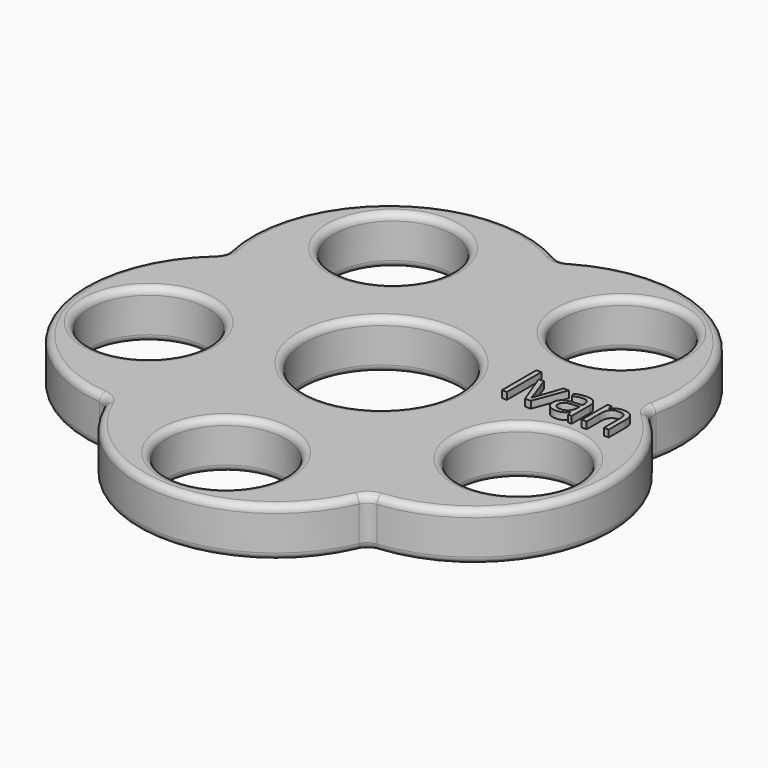
from build123d import *

# Parameters (mm, degrees)
F0_R         = 8.5
F0_R_2       = 11
F1_DEPTH     = 7
F2_R         = 2
F3_R         = 1
F4_TEXT_SIZE = 8.692171347
F5_DEPTH     = 1


# Not quite as in the source:
# - Text() gives the source's letters only with a copy of the font that has no kerning and outlines rounded to 1/6400 em; it was checked with that copy


with BuildPart() as f1:
    # F0 (on Top) → F1 (new body)
    with BuildSketch(Plane.XY):
        with BuildLine():
            ThreePointArc((30.3984422568, 9.877052624), (22.9236248394, 31.5516627806), (0, 31.9628137087))
            ThreePointArc((0, 31.9628137087), (-22.9236248394, 31.5516627806), (-30.3984422568, 9.877052624))
            ThreePointArc((-30.3984422568, 9.877052624), (-37.0912041355, -12.0516627806), (-18.7872705198, -25.8584594784))
            ThreePointArc((-18.7872705198, -25.8584594784), (0, -39), (18.7872705198, -25.8584594784))
            ThreePointArc((18.7872705198, -25.8584594784), (37.0912041355, -12.0516627806), (30.3984422568, 9.877052624))
        make_face()
        with Locations((0, -28)):
            Circle(F0_R, mode=Mode.SUBTRACT)
        with Locations((-26.6295824563, -8.6524758425)):
            Circle(F0_R, mode=Mode.SUBTRACT)
        with Locations((26.6295824563, -8.6524758425)):
            Circle(F0_R, mode=Mode.SUBTRACT)
        Circle(F0_R_2, mode=Mode.SUBTRACT)
        with Locations((-16.4579870642, 22.6524758425)):
            Circle(F0_R, mode=Mode.SUBTRACT)
        with Locations((16.4579870642, 22.6524758425)):
            Circle(F0_R, mode=Mode.SUBTRACT)
    extrude(amount=F1_DEPTH)

    # F2
    f2_edges = [f1.edges().sort_by_distance(p)[0] for p in [
        (18.787271, -25.858459, 3.5),
        (30.398442, 9.877053, 3.5),
        (0, 31.962814, 3.5),
        (-30.398442, 9.877053, 3.5),
        (-18.787271, -25.858459, 3.5),
    ]]
    fillet(f2_edges, radius=F2_R)

    # F3
    f3_edges = [f1.edges().sort_by_distance(p)[0] for p in [
        (0, -39, 7),
        (-19.000712, -26.152236, 7),
        (19.000712, -26.152236, 7),
        (-37.091204, -12.051663, 7),
        (37.091204, -12.051663, 7),
        (-30.743797, 9.989265, 7),
        (30.743797, 9.989265, 7),
        (-22.923625, 31.551663, 7),
        (22.923625, 31.551663, 7),
        (0, 32.325942, 7),
        (-8.5, -28, 7),
        (-35.129582, -8.652476, 7),
        (18.129582, -8.652476, 7),
        (-11, 0, 7),
        (-24.957987, 22.652476, 7),
        (7.957987, 22.652476, 7),
        (0, -39, 0),
        (-19.000712, -26.152236, 0),
        (19.000712, -26.152236, 0),
        (-37.091204, -12.051663, 0),
        (37.091204, -12.051663, 0),
        (-30.743797, 9.989265, 0),
        (30.743797, 9.989265, 0),
        (-22.923625, 31.551663, 0),
        (22.923625, 31.551663, 0),
        (0, 32.325942, 0),
        (-8.5, -28, 0),
        (-35.129582, -8.652476, 0),
        (18.129582, -8.652476, 0),
        (-11, 0, 0),
        (-24.957987, 22.652476, 0),
        (7.957987, 22.652476, 0),
    ]]
    fillet(f3_edges, radius=F3_R)

    # F4 (on face) → F5 (join)
    with BuildSketch(Plane.XY.offset(7)):
        with Locations((15.0883411989, 1.7613614909)):
            Text('Ivan', F4_TEXT_SIZE, font='Open Sans', text_align=(TextAlign.LEFT, TextAlign.BOTTOM))
    extrude(amount=F5_DEPTH)


solid = f1.part
